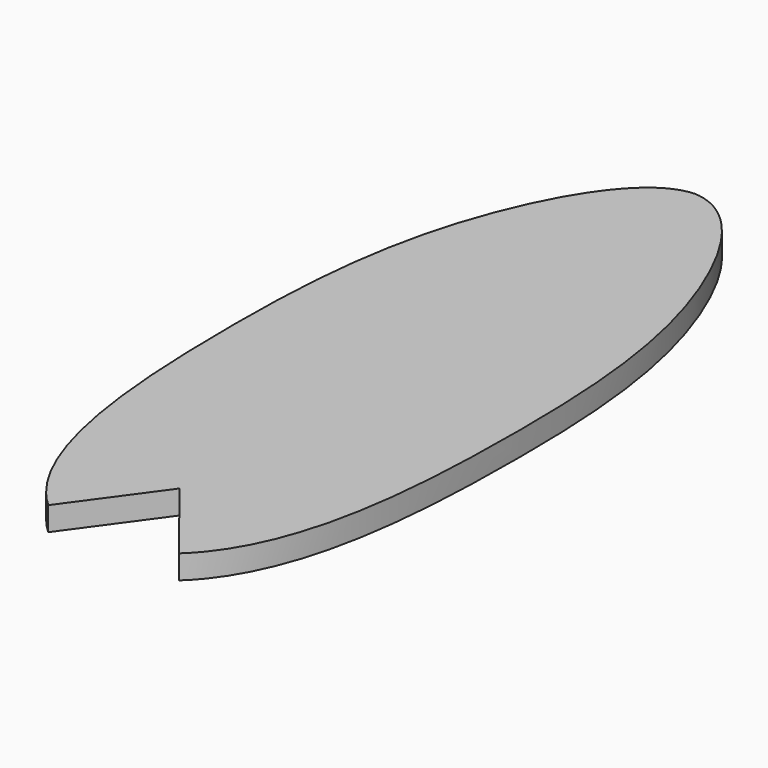
from build123d import *

# Parameters (mm, degrees)
F1_DEPTH = 12.7


with BuildPart() as f1:
    # F0 (on Top) → F1 (new body)
    with BuildSketch(Plane.XY):
        with BuildLine():
            add(Edge.make_bspline(
                [(-479.7950591739, 239.7340460338), (-456.2803178135, 238.7381201493), (-408.8596973192, 159.102307152), (-399.5119730208, 23.5090383581), (-409.1910165745, -115.0536707693), (-444.9865966458, -147.8002653918)],
                knots=[0, 0, 0, 0, 0.1189079678, 0.2727344342, 0.4346446811, 0.4346446811, 0.4346446811, 0.4346446811], degree=3))
            add(Edge.make_bspline(
                [(-479.795059174, 239.7340460338), (-503.3098005344, 238.7381201493), (-550.7304210286, 159.102307152), (-560.0781453271, 23.5090383581), (-550.3991017734, -115.0536707693), (-514.603521702, -147.8002653918)],
                knots=[0, 0, 0, 0, 0.1189079678, 0.2727344342, 0.4346446811, 0.4346446811, 0.4346446811, 0.4346446811], degree=3))
            Line((-514.603521702, -147.8002653918), (-481.2892675399, -101.8401682377))
            Line((-481.2892675399, -101.8401682377), (-444.9865966458, -147.8002653918))
        make_face()
    extrude(amount=F1_DEPTH)


solid = f1.part
